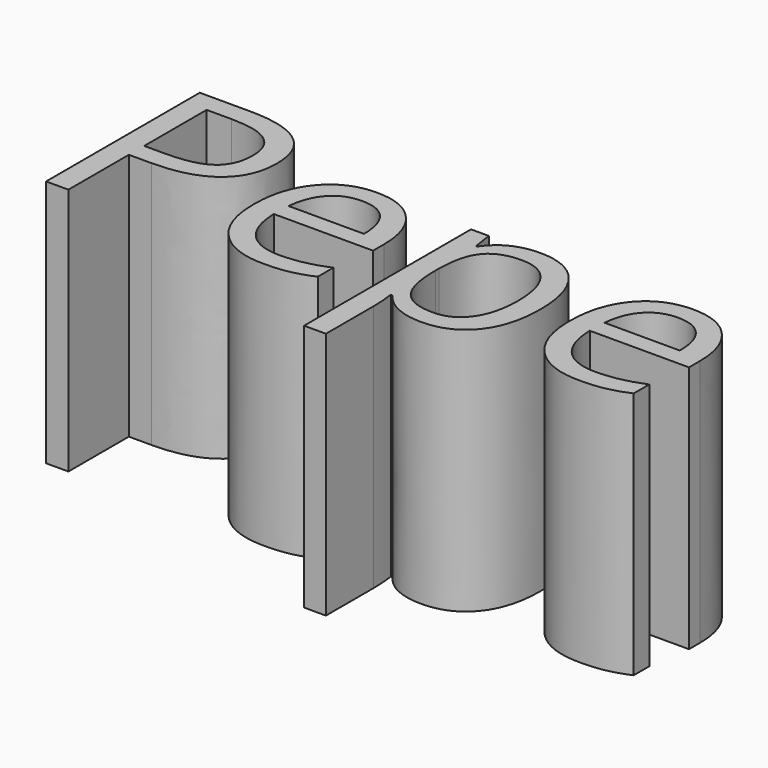
from build123d import *

# Parameters (mm, degrees)
F0_TEXT_SIZE = 32.534696705
F1_DEPTH     = 30


# Not quite as in the source:
# - Text() gives the source's letters only with a copy of the font that has no kerning and outlines rounded to 1/6400 em; it was checked with that copy


with BuildPart() as f1:
    # F0 (on Top) → F1 (new body)
    with BuildSketch(Plane.XY):
        with Locations((-31.0304947197, 5.4759695195)):
            Text('Pepe', F0_TEXT_SIZE, font='Open Sans', text_align=(TextAlign.LEFT, TextAlign.BOTTOM))
    extrude(amount=F1_DEPTH)


solid = f1.part
